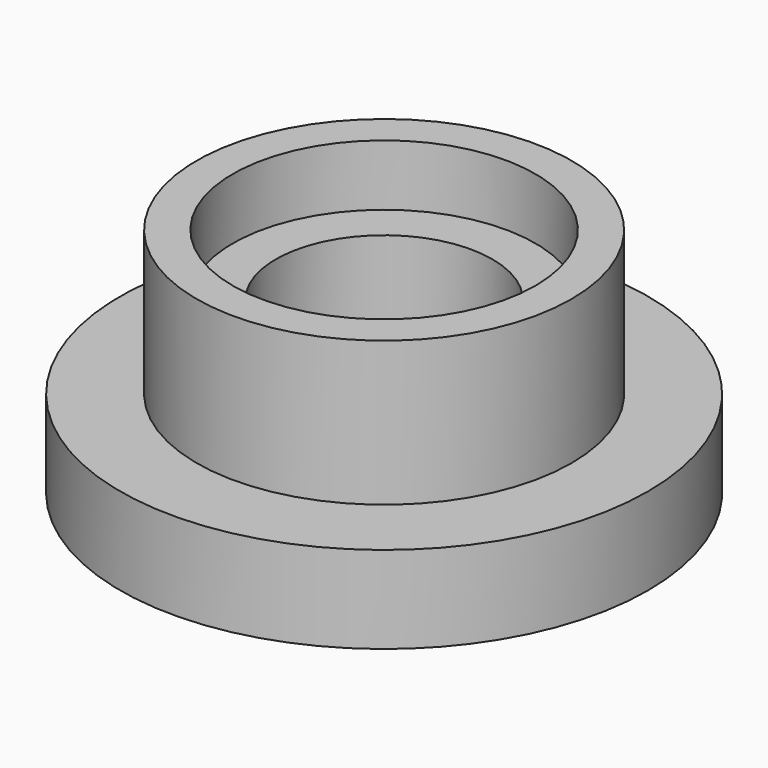
from build123d import *

# Parameters (mm, degrees)
F0_R          = 9.505
F0_R_2        = 8.26
F1_DEPTH      = 3.14
F0_R_3        = 6.75
F0_R_4        = 5.45
F2_DEPTH      = 5.2
F2_DEPTH_BACK = 1
F0_R_5        = 3.9
F3_DEPTH      = 3
F3_DEPTH_BACK = 1
F4_DEPTH      = 1


with BuildPart() as f1:
    # F0 (on Top) → F1 (new body)
    with BuildSketch(Plane.XY):
        Circle(F0_R)
        Circle(F0_R_2, mode=Mode.SUBTRACT)
    extrude(amount=-F1_DEPTH)

    # F0 (on Top) → F4 (join)
    with BuildSketch(Plane.XY):
        Circle(F0_R_2)
        Circle(F0_R_3, mode=Mode.SUBTRACT)
    extrude(amount=-F4_DEPTH)


with BuildPart() as f2:
    # F0 (on Top) → F2 (new body, two sides)
    with BuildSketch(Plane.XY) as f2_sk:
        Circle(F0_R_3)
        Circle(F0_R_4, mode=Mode.SUBTRACT)
    extrude(amount=F2_DEPTH)
    extrude(f2_sk.sketch, amount=-F2_DEPTH_BACK)

    # F0 (on Top) → F3 (join, two sides)
    with BuildSketch(Plane.XY) as f3_sk:
        Circle(F0_R_4)
        Circle(F0_R_5, mode=Mode.SUBTRACT)
    extrude(amount=F3_DEPTH)
    extrude(f3_sk.sketch, amount=-F3_DEPTH_BACK)


with BuildPart() as f4:
    # F0 (on Top) → F4, piece 2 (new body)
    with BuildSketch(Plane.XY):
        Circle(F0_R_5)
    extrude(amount=-F4_DEPTH)


solid = Compound([f1.part, f2.part, f4.part])
